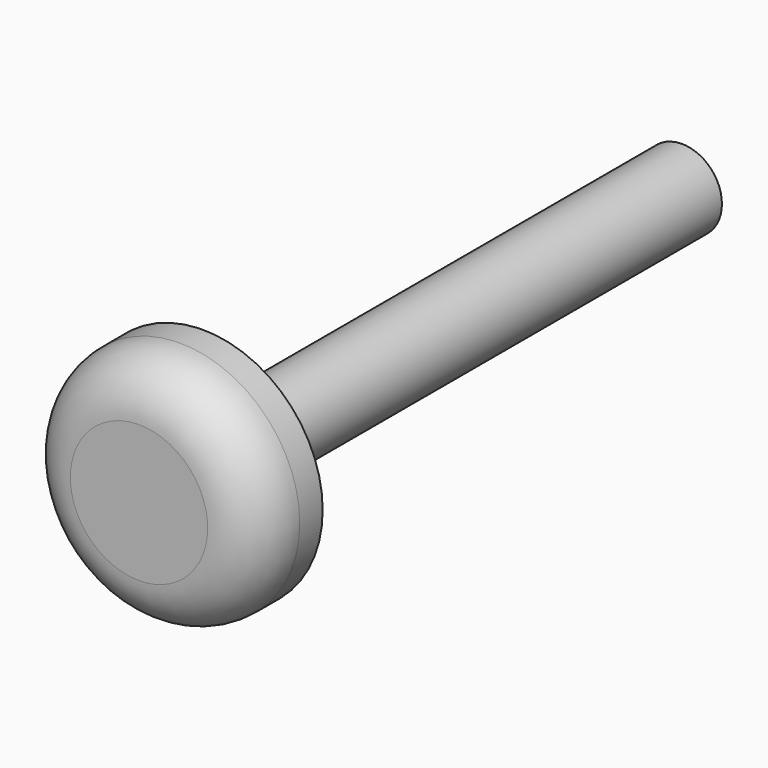
from build123d import *

# Parameters (mm, degrees)
F0_R     = 1.5875
F1_DEPTH = 11.90625
F2_R     = 4.7625
F3_DEPTH = 3.175
F4_R     = 2.032


# Not quite as in the source:
# - a length typed as a fraction of an inch, garbled in the dataset ("3 / 203.2 mm" for 3/8 in), is restored


with BuildPart() as f1:
    # F0 (on Front) → F1 (new body, symmetric)
    with BuildSketch(Plane.XZ):
        Circle(F0_R)
    extrude(amount=F1_DEPTH, both=True)

    # F2 (on face) → F3 (join)
    with BuildSketch(Plane.XZ.offset(11.90625)):
        Circle(F2_R)
    extrude(amount=F3_DEPTH)

    # F4
    f4_edges = [f1.edges().sort_by_distance(p)[0] for p in [
        (-4.7625, -15.08125, 0),
    ]]
    fillet(f4_edges, radius=F4_R)


solid = f1.part
